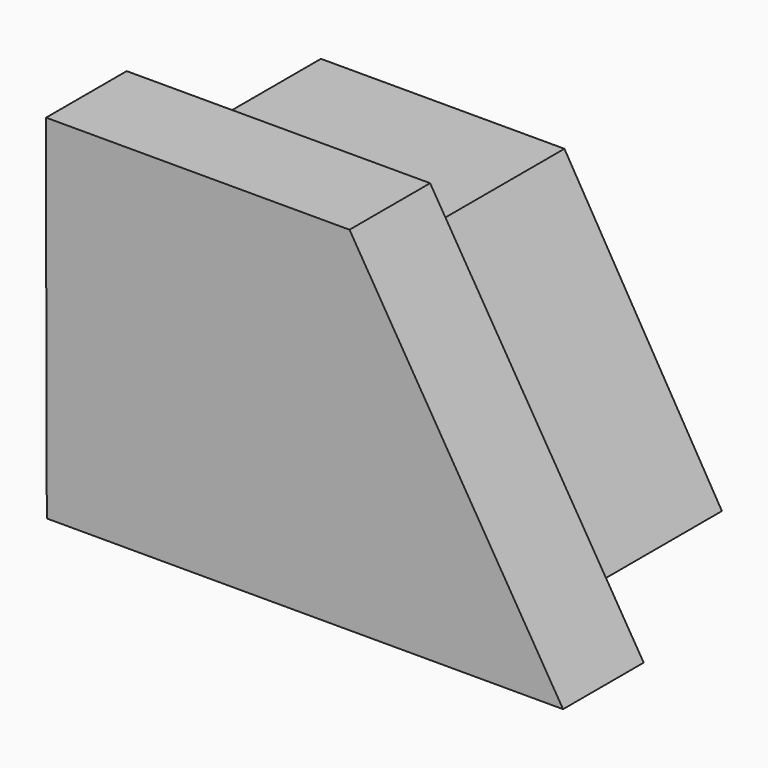
from build123d import *

# Parameters (mm, degrees)
F1_DEPTH = 61.214
F3_DEPTH = 25.4


with BuildPart() as f1:
    # F0 (on Front) → F1 (new body)
    with BuildSketch(Plane.XZ):
        Polygon((-15.1163935661, 27.3316595703), (-76.4981135726, 27.3316595703), (-76.1927291751, -40.1576943696), (24.5832242072, -40.1576943696), align=None)
    extrude(amount=-F1_DEPTH)


with BuildPart() as f3:
    # F2 (on Front) → F3 (new body)
    with BuildSketch(Plane.XZ):
        Polygon((-76.4930769801, 49.4907200336), (-76.4930769801, 27.311546728), (-76.3097777963, -39.409276098), (53.8324899971, -39.409276098), (0, 49.4907200336), align=None)
    extrude(amount=F3_DEPTH)


solid = Compound([f1.part, f3.part])
